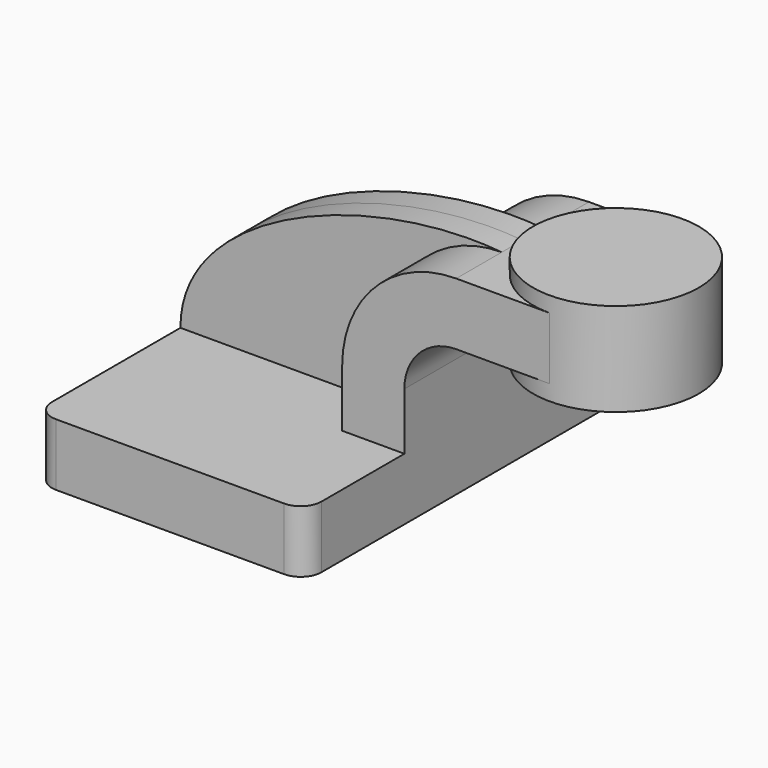
from build123d import *

# Parameters (mm, degrees)
F1_DEPTH = 2.5
F0_W     = 1
F0_H     = 0.75
F2_DEPTH = 1
F3_DEPTH = 0.3125
F5_R     = 0.25


with BuildPart() as f1:
    # F0 (on Front) → F1 (new body, symmetric)
    with BuildSketch(Plane.XZ):
        Polygon((-1.625, 0.375), (-1.625, -0.375), (1.625, -0.375), (1.625, 0.375), (0.875, 0.375), align=None)
    extrude(amount=F1_DEPTH, both=True)

    # F0 (on Front) → F2 (join, symmetric)
    with BuildSketch(Plane.XZ):
        with BuildLine():
            Line((0.875, 0.375), (1.625, 0.375))
            Line((1.625, 0.375), (1.625, 1.063))
            ThreePointArc((1.625, 1.063), (1.8080582618, 1.5049417382), (2.25, 1.688))
            Line((2.25, 1.688), (2.375, 1.688))
            Line((2.375, 1.688), (2.375, 2.438))
            Line((2.375, 2.438), (2.25, 2.438))
            ThreePointArc((2.25, 2.438), (1.2777281759, 2.0352718241), (0.875, 1.063))
            Line((0.875, 1.063), (0.875, 0.375))
        make_face()
        with Locations((2.875, 2.063)):
            Rectangle(F0_W, F0_H)
    extrude(amount=F2_DEPTH, both=True)

    # F0 (on Front) → F3 (join, symmetric)
    with BuildSketch(Plane.XZ):
        with BuildLine():
            add(Edge.make_bspline(
                [(-1.625, 0.375), (-1.6311762156, 1.7044375418), (0.6304873386, 2.588064177), (2.25, 2.438)],
                knots=[0, 0, 0, 0, 4.3899423686, 4.3899423686, 4.3899423686, 4.3899423686], degree=3))
            Line((-1.625, 0.375), (0.875, 0.375))
            Line((0.875, 0.375), (0.875, 1.063))
            ThreePointArc((0.875, 1.063), (1.2777281759, 2.0352718241), (2.25, 2.438))
        make_face()
    extrude(amount=F3_DEPTH, both=True)

    # F0 (on Front) → F4 (revolve)
    with BuildSketch(Plane.XZ):
        Polygon((3.375, 2.625), (3.375, 2.438), (3.375, 1.688), (3.375, 1.5), (4.375, 1.5), (4.375, 2.625), align=None)
    revolve(axis=Axis((3.375, 0, 2.0625), (0, 0, 1)))

    # F5
    f5_edges = [f1.edges().sort_by_distance(p)[0] for p in [
        (1.625, -2.5, 0),
        (-1.625, -2.5, 0),
        (-1.625, 2.5, 0),
        (1.625, 2.5, 0),
    ]]
    fillet(f5_edges, radius=F5_R)


solid = f1.part
